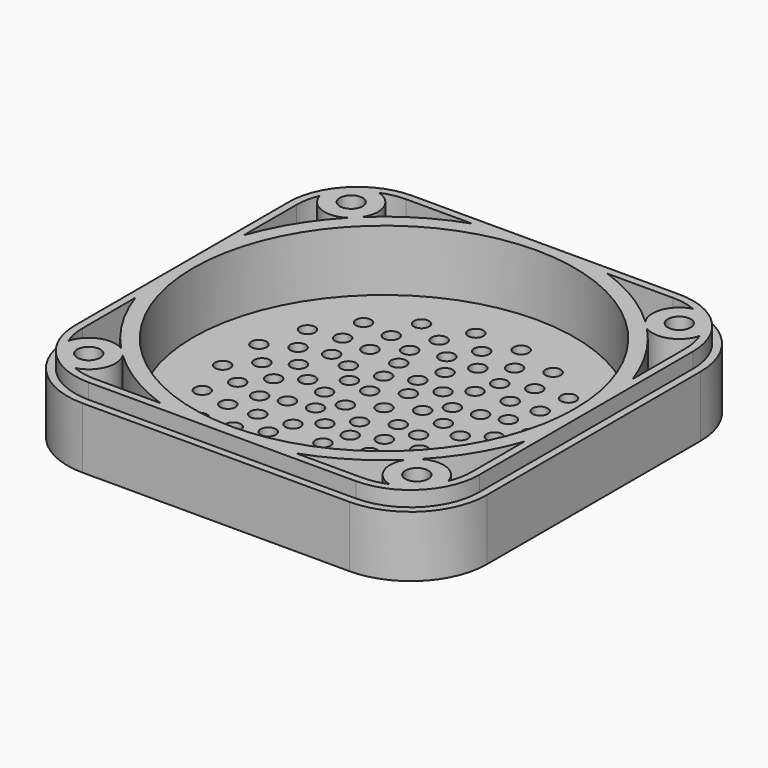
from build123d import *

# Parameters (mm, degrees)
F1_DEPTH  = 10
F2_R      = 1
F3_DEPTH  = 10.001
F4_R      = 25
F5_DEPTH  = 8
F6_R      = 1.5
F7_DEPTH  = 10.001
F8_T      = 2
F9_SIZE2  = 2
F9_SIZE   = 2
F11_DEPTH = 2


# Not quite as in the source:
# - a shell that OpenCascade refuses in one call is made with other operations: the cavity is built on its own and cut out


with BuildPart() as f1:
    # F0 (on Top) → F1 (new body)
    with BuildSketch(Plane.XY):
        with BuildLine():
            Line((-17.5, -27.5), (17.5, -27.5))
            ThreePointArc((17.5, -27.5), (24.5710678119, -24.5710678119), (27.5, -17.5))
            Line((27.5, -17.5), (27.5, 17.5))
            ThreePointArc((27.5, 17.5), (24.5710678119, 24.5710678119), (17.5, 27.5))
            Line((17.5, 27.5), (-17.5, 27.5))
            ThreePointArc((-17.5, 27.5), (-24.5710678119, 24.5710678119), (-27.5, 17.5))
            Line((-27.5, 17.5), (-27.5, -17.5))
            ThreePointArc((-27.5, -17.5), (-24.5710678119, -24.5710678119), (-17.5, -27.5))
        make_face()
    extrude(amount=F1_DEPTH)

    # F2 (on face) → F3 (cut, through all)
    with BuildSketch(Plane.XY.offset(10)):
        with Locations((8.6602540378, 5)):
            Circle(F2_R)
        with Locations((-9.1923881554, -9.1923881554)):
            Circle(F2_R)
        with Locations((12.8399484277, -2.0336480455)):
            Circle(F2_R)
        with Locations((13.4350288425, -13.4350288425)):
            Circle(F2_R)
        with Locations((-5.9018764966, 11.5830848144)):
            Circle(F2_R)
        with Locations((-12.94427191, -9.4045640367)):
            Circle(F2_R)
        with Locations((-16.9291239596, 8.6258194951)):
            Circle(F2_R)
        with Locations((16.9291239596, -8.6258194951)):
            Circle(F2_R)
        with Locations((9.1923881554, 9.1923881554)):
            Circle(F2_R)
        with Locations((18.7660784713, -2.9722548358)):
            Circle(F2_R)
        with Locations((4.4052427373, -5.4400217302)):
            Circle(F2_R)
        with Locations((-15.2169042607, 4.94427191)):
            Circle(F2_R)
        with Locations((0, 16)):
            Circle(F2_R)
        with Locations((-3.4641016151, 2)):
            Circle(F2_R)
        with Locations((15.2169042607, -4.94427191)):
            Circle(F2_R)
        with Locations((3.4641016151, -2)):
            Circle(F2_R)
        with Locations((-18.7660784713, 2.9722548358)):
            Circle(F2_R)
        with Locations((-10, 0)):
            Circle(F2_R)
        with Locations((12.94427191, 9.4045640367)):
            Circle(F2_R)
        with Locations((-18.7660784713, -2.9722548358)):
            Circle(F2_R)
        with Locations((-16.9291239596, -8.6258194951)):
            Circle(F2_R)
        with Locations((0, 10)):
            Circle(F2_R)
        with Locations((-13.4350288425, -13.4350288425)):
            Circle(F2_R)
        with Locations((2.9722548358, -18.7660784713)):
            Circle(F2_R)
        with Locations((-2.9722548358, -18.7660784713)):
            Circle(F2_R)
        with Locations((-8.6258194951, -16.9291239596)):
            Circle(F2_R)
        with Locations((8.6258194951, -16.9291239596)):
            Circle(F2_R)
        with Locations((-4.4052427373, 5.4400217302)):
            Circle(F2_R)
        with Locations((6.5350629855, -2.5085756468)):
            Circle(F2_R)
        with Locations((12.94427191, -9.4045640367)):
            Circle(F2_R)
        with Locations((-8.6602540378, -5)):
            Circle(F2_R)
        with Locations((-5.4400217302, -4.4052427373)):
            Circle(F2_R)
        with Locations((2.5085756468, 6.5350629855)):
            Circle(F2_R)
        with Locations((-8.6258194951, 16.9291239596)):
            Circle(F2_R)
        with Locations((5, -8.6602540378)):
            Circle(F2_R)
        with Locations((5.9018764966, -11.5830848144)):
            Circle(F2_R)
        with Locations((8.6258194951, 16.9291239596)):
            Circle(F2_R)
        with Locations((5.9018764966, 11.5830848144)):
            Circle(F2_R)
        with Locations((-6.5350629855, 2.5085756468)):
            Circle(F2_R)
        with Locations((-5.9018764966, -11.5830848144)):
            Circle(F2_R)
        with Locations((-3.4641016151, -2)):
            Circle(F2_R)
        with Locations((-11.5830848144, -5.9018764966)):
            Circle(F2_R)
        with Locations((11.5830848144, -5.9018764966)):
            Circle(F2_R)
        with Locations((5, 8.6602540378)):
            Circle(F2_R)
        with Locations((0, -16)):
            Circle(F2_R)
        with Locations((10, 0)):
            Circle(F2_R)
        with Locations((-8.6602540378, 5)):
            Circle(F2_R)
        with Locations((-12.8399484277, 2.0336480455)):
            Circle(F2_R)
        with Locations((12.8399484277, 2.0336480455)):
            Circle(F2_R)
        with Locations((-4.94427191, 15.2169042607)):
            Circle(F2_R)
        with Locations((1.0950412553, -6.9138183842)):
            Circle(F2_R)
        with Locations((-9.1923881554, 9.1923881554)):
            Circle(F2_R)
        with Locations((-9.4045640367, -12.94427191)):
            Circle(F2_R)
        with Locations((-16, 0)):
            Circle(F2_R)
        with Locations((-12.94427191, 9.4045640367)):
            Circle(F2_R)
        with Locations((4.94427191, 15.2169042607)):
            Circle(F2_R)
        with Locations((9.4045640367, -12.94427191)):
            Circle(F2_R)
        with Locations((16, 0)):
            Circle(F2_R)
        with Locations((2.9722548358, 18.7660784713)):
            Circle(F2_R)
        with Locations((6.9138183842, 1.0950412553)):
            Circle(F2_R)
        with Locations((-4.94427191, -15.2169042607)):
            Circle(F2_R)
        with Locations((-11.5830848144, 5.9018764966)):
            Circle(F2_R)
        with Locations((-5, -8.6602540378)):
            Circle(F2_R)
        with Locations((-2.0336480455, -12.8399484277)):
            Circle(F2_R)
        with Locations((2.0336480455, 12.8399484277)):
            Circle(F2_R)
        with Locations((-6.9138183842, -1.0950412553)):
            Circle(F2_R)
        with Locations((-13.4350288425, 13.4350288425)):
            Circle(F2_R)
        with Locations((16.9291239596, 8.6258194951)):
            Circle(F2_R)
        with Locations((18.7660784713, 2.9722548358)):
            Circle(F2_R)
        with Locations((2.0336480455, -12.8399484277)):
            Circle(F2_R)
        with Locations((13.4350288425, 13.4350288425)):
            Circle(F2_R)
        with Locations((0, -10)):
            Circle(F2_R)
        with Locations((5.4400217302, 4.4052427373)):
            Circle(F2_R)
        with Locations((-2.9722548358, 18.7660784713)):
            Circle(F2_R)
        with Locations((15.2169042607, 4.94427191)):
            Circle(F2_R)
        with Locations((0, -4)):
            Circle(F2_R)
        with Locations((-15.2169042607, -4.94427191)):
            Circle(F2_R)
        with Locations((-2.0336480455, 12.8399484277)):
            Circle(F2_R)
        with Locations((-1.0950412553, 6.9138183842)):
            Circle(F2_R)
        with Locations((11.5830848144, 5.9018764966)):
            Circle(F2_R)
        with Locations((3.4641016151, 2)):
            Circle(F2_R)
        with Locations((9.4045640367, 12.94427191)):
            Circle(F2_R)
        with Locations((4.94427191, -15.2169042607)):
            Circle(F2_R)
        with Locations((-9.4045640367, 12.94427191)):
            Circle(F2_R)
        with Locations((-2.5085756468, -6.5350629855)):
            Circle(F2_R)
        with Locations((0, 4)):
            Circle(F2_R)
        with Locations((-5, 8.6602540378)):
            Circle(F2_R)
        with Locations((8.6602540378, -5)):
            Circle(F2_R)
        with Locations((9.1923881554, -9.1923881554)):
            Circle(F2_R)
        with Locations((-12.8399484277, -2.0336480455)):
            Circle(F2_R)
        Circle(F2_R)
    extrude(amount=-F3_DEPTH, mode=Mode.SUBTRACT)

    # F4 (on face) → F5 (cut)
    with BuildSketch(Plane.XY.offset(10)):
        Circle(F4_R)
    extrude(amount=-F5_DEPTH, mode=Mode.SUBTRACT)

    # F6 (on face) → F7 (cut, through all)
    with BuildSketch(Plane.XY.offset(10)):
        with Locations((-21.5, 21.5)):
            Circle(F6_R)
        with Locations((21.5, 21.5)):
            Circle(F6_R)
        with Locations((21.5, -21.5)):
            Circle(F6_R)
        with Locations((-21.5, -21.5)):
            Circle(F6_R)
    extrude(amount=-F7_DEPTH, mode=Mode.SUBTRACT)

    # F8: shell of thickness 2, made by hand


with BuildPart() as f8_core1:
    # F8_t2: copy of F1
    add(f1.part)

    # the walls: a layer under each face that stays
    f8_faces = [f8_core1.faces().sort_by_distance(p)[0] for p in [
        (0, -27.5, 5),
        (-24.5710678119, -24.5710678119, 5),
        (24.5710678119, -24.5710678119, 5),
        (-18.3333333333, -18.3333333333, 0),
        (-27.5, 0, 5),
        (27.5, 0, 5),
        (-24.5710678119, 24.5710678119, 5),
        (24.5710678119, 24.5710678119, 5),
        (0, 27.5, 5),
        (-23, -21.5, 5),
        (-14.4350288425, -13.4350288425, 1),
        (-3.9722548358, -18.7660784713, 1),
        (-9.6258194951, -16.9291239596, 1),
        (-10.4045640367, -12.94427191, 1),
        (-6.9018764966, -11.5830848144, 1),
        (-5.94427191, -15.2169042607, 1),
        (-3.0336480455, -12.8399484277, 1),
        (-17.9291239596, -8.6258194951, 1),
        (-13.94427191, -9.4045640367, 1),
        (-12.5830848144, -5.9018764966, 1),
        (-19.7660784713, -2.9722548358, 1),
        (-16.2169042607, -4.94427191, 1),
        (-13.8399484277, -2.0336480455, 1),
        (-10.1923881554, -9.1923881554, 1),
        (-6, -8.6602540378, 1),
        (-3.5085756468, -6.5350629855, 1),
        (-9.6602540378, -5, 1),
        (-7.9138183842, -1.0950412553, 1),
        (-6.4400217302, -4.4052427373, 1),
        (-4.4641016151, -2, 1),
        (1.9722548358, -18.7660784713, 1),
        (-1, -16, 1),
        (3.94427191, -15.2169042607, 1),
        (1.0336480455, -12.8399484277, 1),
        (7.6258194951, -16.9291239596, 1),
        (4.9018764966, -11.5830848144, 1),
        (8.4045640367, -12.94427191, 1),
        (20, -21.5, 5),
        (12.4350288425, -13.4350288425, 1),
        (-1, -10, 1),
        (4, -8.6602540378, 1),
        (0.0950412553, -6.9138183842, 1),
        (8.1923881554, -9.1923881554, 1),
        (-1, -4, 1),
        (3.4052427373, -5.4400217302, 1),
        (2.4641016151, -2, 1),
        (7.6602540378, -5, 1),
        (5.5350629855, -2.5085756468, 1),
        (11.94427191, -9.4045640367, 1),
        (15.9291239596, -8.6258194951, 1),
        (10.5830848144, -5.9018764966, 1),
        (14.2169042607, -4.94427191, 1),
        (11.8399484277, -2.0336480455, 1),
        (17.7660784713, -2.9722548358, 1),
        (-19.7660784713, 2.9722548358, 1),
        (-17, 0, 1),
        (-13.8399484277, 2.0336480455, 1),
        (-16.2169042607, 4.94427191, 1),
        (-12.5830848144, 5.9018764966, 1),
        (-17.9291239596, 8.6258194951, 1),
        (-13.94427191, 9.4045640367, 1),
        (-11, 0, 1),
        (-7.5350629855, 2.5085756468, 1),
        (-9.6602540378, 5, 1),
        (-4.4641016151, 2, 1),
        (-5.4052427373, 5.4400217302, 1),
        (-10.1923881554, 9.1923881554, 1),
        (-2.0950412553, 6.9138183842, 1),
        (-6, 8.6602540378, 1),
        (-14.4350288425, 13.4350288425, 1),
        (-23, 21.5, 5),
        (-10.4045640367, 12.94427191, 1),
        (-6.9018764966, 11.5830848144, 1),
        (-9.6258194951, 16.9291239596, 1),
        (-3.0336480455, 12.8399484277, 1),
        (-5.94427191, 15.2169042607, 1),
        (-3.9722548358, 18.7660784713, 1),
        (-1, 0, 1),
        (2.4641016151, 2, 1),
        (-1, 4, 1),
        (4.4400217302, 4.4052427373, 1),
        (5.9138183842, 1.0950412553, 1),
        (9, 0, 1),
        (7.6602540378, 5, 1),
        (1.5085756468, 6.5350629855, 1),
        (-1, 10, 1),
        (4, 8.6602540378, 1),
        (8.1923881554, 9.1923881554, 1),
        (11.8399484277, 2.0336480455, 1),
        (15, 0, 1),
        (14.2169042607, 4.94427191, 1),
        (17.7660784713, 2.9722548358, 1),
        (10.5830848144, 5.9018764966, 1),
        (11.94427191, 9.4045640367, 1),
        (15.9291239596, 8.6258194951, 1),
        (1.0336480455, 12.8399484277, 1),
        (-1, 16, 1),
        (3.94427191, 15.2169042607, 1),
        (4.9018764966, 11.5830848144, 1),
        (8.4045640367, 12.94427191, 1),
        (7.6258194951, 16.9291239596, 1),
        (1.9722548358, 18.7660784713, 1),
        (12.4350288425, 13.4350288425, 1),
        (20, 21.5, 5),
        (-25, 0, 6),
        (-16.6666666667, -16.6666666667, 2),
    ]]
    thicken(f8_faces, amount=-F8_T, mode=Mode.SUBTRACT)

    # F8_s3 → F8_t4 (revolve, cut)
    with BuildSketch(Plane.XZ):
        Polygon((24.98, 2.02), (27, 2), (27, 0), (25, 0), align=None)
    revolve(axis=Axis((0, 0, 2), (0, 0, 1)), mode=Mode.SUBTRACT)


with BuildPart() as f1_1:
    add(f1.part)

    # what is left inside the walls is the cavity
    f8_cavity = [f8_core1.part.solids().sort_by_distance(p)[0] for p in [
        (-14.03206, -23.090727, 4.666667),
        (14.03206, -23.090727, 4.666667),
        (-23.090727, -14.03206, 4.666667),
        (23.090727, -14.03206, 4.666667),
        (-23.090727, 14.03206, 4.666667),
        (-14.03206, 23.090727, 4.666667),
        (14.03206, 23.090727, 4.666667),
        (23.090727, 14.03206, 4.666667),
    ]]
    add(f8_cavity, mode=Mode.SUBTRACT)

    # F9
    f9_edges = [f1_1.edges().sort_by_distance(p)[0] for p in [
        (20, 21.5, 0),
        (-23, 21.5, 0),
        (-23, -21.5, 0),
        (20, -21.5, 0),
    ]]
    chamfer(f9_edges, length=F9_SIZE, length2=F9_SIZE2)

    # F10 (on face) → F11 (cut)
    with BuildSketch(Plane.XY.offset(10)):
        with BuildLine():
            ThreePointArc((-27.5, -17.5), (-24.5710678119, -24.5710678119), (-17.5, -27.5))
            Line((-17.5, -27.5), (17.5, -27.5))
            ThreePointArc((17.5, -27.5), (24.5710678119, -24.5710678119), (27.5, -17.5))
            Line((27.5, -17.5), (27.5, 17.5))
            ThreePointArc((27.5, 17.5), (24.5710678119, 24.5710678119), (17.5, 27.5))
            Line((17.5, 27.5), (-17.5, 27.5))
            ThreePointArc((-17.5, 27.5), (-24.5710678119, 24.5710678119), (-27.5, 17.5))
            Line((-27.5, 17.5), (-27.5, -17.5))
        make_face()
        with BuildLine():
            Line((-17.5, 26.5), (17.5, 26.5))
            ThreePointArc((17.5, 26.5), (23.8639610307, 23.8639610307), (26.5, 17.5))
            Line((26.5, 17.5), (26.5, -17.5))
            ThreePointArc((26.5, -17.5), (23.8639610307, -23.8639610307), (17.5, -26.5))
            Line((17.5, -26.5), (-17.5, -26.5))
            ThreePointArc((-17.5, -26.5), (-23.8639610307, -23.8639610307), (-26.5, -17.5))
            Line((-26.5, -17.5), (-26.5, 17.5))
            ThreePointArc((-26.5, 17.5), (-23.8639610307, 23.8639610307), (-17.5, 26.5))
        make_face(mode=Mode.SUBTRACT)
    extrude(amount=-F11_DEPTH, mode=Mode.SUBTRACT)


solid = f1_1.part
